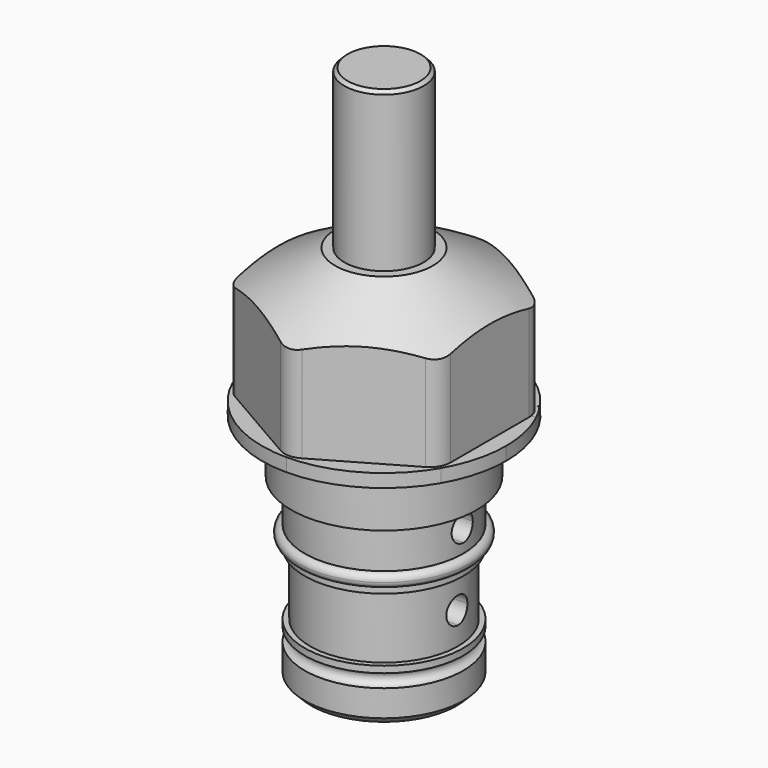
from build123d import *

# Parameters (mm, degrees)
F0_R     = 7.9375
F1_DEPTH = 35.56
F2_DEPTH = 3.175
F3_R     = 5.08
F7_SIZE  = 1.5875
F9_DEPTH = 29.3303937748
F10_W    = 9.525
F10_H    = 37.465
F10_W_2  = 3.175
F10_W_3  = 12.7
F10_H_2  = 22.606
F13_SIZE = 0.79375


with BuildPart() as f1:
    # F0 (on Top) → F1 (new body)
    with BuildSketch(Plane.XY):
        Polygon((25.4, -14.6646968374), (25.4, 14.6646968374), (0, 29.3293936748), (-25.4, 14.6646968374), (-25.4, -14.6646968374), (0, -29.3293936748), align=None)
        Circle(F0_R, mode=Mode.SUBTRACT)
        Circle(F0_R)
    extrude(amount=F1_DEPTH)

    # F0 (on Top) → F2 (join)
    with BuildSketch(Plane.XY):
        with BuildLine():
            ThreePointArc((-25.4, -14.6646968374), (-14.6646968374, -25.4), (0, -29.3293936748))
            Line((0, -29.3293936748), (-25.4, -14.6646968374))
        make_face()
        with BuildLine():
            ThreePointArc((0, -29.3293936748), (14.6646968374, -25.4), (25.4, -14.6646968374))
            Line((25.4, -14.6646968374), (0, -29.3293936748))
        make_face()
        with BuildLine():
            ThreePointArc((25.4, -14.6646968374), (28.3300188199, -7.5910056644), (29.3293936748, 0))
            ThreePointArc((29.3293936748, 0), (28.3300188199, 7.5910056644), (25.4, 14.6646968374))
            Line((25.4, 14.6646968374), (25.4, -14.6646968374))
        make_face()
        Polygon((25.4, -14.6646968374), (25.4, 14.6646968374), (0, 29.3293936748), (-25.4, 14.6646968374), (-25.4, -14.6646968374), (0, -29.3293936748), align=None)
        Circle(F0_R, mode=Mode.SUBTRACT)
        with BuildLine():
            Line((0, 29.3293936748), (25.4, 14.6646968374))
            ThreePointArc((25.4, 14.6646968374), (14.6646968374, 25.4), (0, 29.3293936748))
        make_face()
        with BuildLine():
            Line((-25.4, 14.6646968374), (0, 29.3293936748))
            ThreePointArc((0, 29.3293936748), (-14.6646968374, 25.4), (-25.4, 14.6646968374))
        make_face()
        with BuildLine():
            Line((-25.4, -14.6646968374), (-25.4, 14.6646968374))
            ThreePointArc((-25.4, 14.6646968374), (-29.3293936748, 0), (-25.4, -14.6646968374))
        make_face()
    extrude(amount=F2_DEPTH)

    # F3 (call 1 of 6: OpenCascade refuses the feature's edges together)
    f3_edges = [f1.edges().sort_by_distance(p)[0] for p in [
        (0, -29.329394, 19.3675),
    ]]
    fillet(f3_edges, radius=F3_R)

    # F3#2 (call 2 of 6)
    f3_2_edges = [f1.edges().sort_by_distance(p)[0] for p in [
        (25.4, -14.664697, 19.3675),
    ]]
    fillet(f3_2_edges, radius=F3_R)

    # F3#3 (call 3 of 6)
    f3_3_edges = [f1.edges().sort_by_distance(p)[0] for p in [
        (25.4, 14.664697, 19.3675),
    ]]
    fillet(f3_3_edges, radius=F3_R)

    # F3#4 (call 4 of 6)
    f3_4_edges = [f1.edges().sort_by_distance(p)[0] for p in [
        (0, 29.329394, 19.3675),
    ]]
    fillet(f3_4_edges, radius=F3_R)

    # F3#5 (call 5 of 6)
    f3_5_edges = [f1.edges().sort_by_distance(p)[0] for p in [
        (-25.4, 14.664697, 19.3675),
    ]]
    fillet(f3_5_edges, radius=F3_R)

    # F3#6 (call 6 of 6)
    f3_6_edges = [f1.edges().sort_by_distance(p)[0] for p in [
        (-25.4, -14.664697, 19.3675),
    ]]
    fillet(f3_6_edges, radius=F3_R)

    # F4 (on Right) → F5 (revolve, cut)
    with BuildSketch(Plane.YZ):
        Polygon((35.3962906179, 35.56), (11.7317574699, 35.56), (35.3962906179, 21.8972754168), align=None)
    revolve(axis=Axis((0, 0, 25.9955581278), (0, 0, -1)), mode=Mode.SUBTRACT)

    # F4 (on Right) → F6 (revolve)
    with BuildSketch(Plane.YZ):
        with BuildLine():
            Line((17.78, -27.686), (0, -27.686))
            Line((0, -27.686), (0, -32.131))
            ThreePointArc((0, -32.131), (2.2450640303, -33.0609359697), (3.175, -35.306))
            ThreePointArc((3.175, -35.306), (2.2450640303, -37.5510640303), (0, -38.481))
            Line((0, -38.481), (0, -42.926))
            Line((0, -42.926), (17.78, -42.926))
            Line((17.78, -42.926), (17.78, -27.686))
        make_face()
        with BuildLine():
            Line((19.05, -12.7), (0, -12.7))
            Line((0, -12.7), (0, -14.2875))
            ThreePointArc((0, -14.2875), (2.2450640303, -15.2174359697), (3.175, -17.4625))
            ThreePointArc((3.175, -17.4625), (2.2450640303, -19.7075640303), (0, -20.6375))
            Line((0, -20.6375), (0, -27.686))
            Line((0, -27.686), (17.78, -27.686))
            Line((17.78, -27.686), (19.05, -27.686))
            Line((19.05, -27.686), (19.05, -26.0985))
            ThreePointArc((19.05, -26.0985), (17.4625, -24.511), (19.05, -22.9235))
            Line((19.05, -22.9235), (19.05, -12.7))
        make_face()
        Polygon((22.225, 0), (0, 0), (0, -12.7), (19.05, -12.7), (22.225, -12.7), align=None)
        with BuildLine():
            Line((19.05, -42.926), (17.78, -42.926))
            Line((17.78, -42.926), (0, -42.926))
            Line((0, -42.926), (0, -55.626))
            Line((0, -55.626), (19.05, -55.626))
            Line((19.05, -55.626), (19.05, -47.6885))
            ThreePointArc((19.05, -47.6885), (17.4625, -46.101), (19.05, -44.5135))
            Line((19.05, -44.5135), (19.05, -42.926))
        make_face()
    revolve(axis=Axis((0, 0, 25.9955581278), (0, 0, -1)))

    # F7
    f7_edges = [f1.edges().sort_by_distance(p)[0] for p in [
        (0, -19.05, -55.626),
    ]]
    chamfer(f7_edges, length=F7_SIZE)


with BuildPart() as f8:
    # F4 (on Right) → F8 (revolve)
    with BuildSketch(Plane.YZ):
        with BuildLine():
            Line((0, -20.6375), (0, -14.2875))
            ThreePointArc((0, -14.2875), (-3.175, -17.4625), (0, -20.6375))
        make_face()
    revolve(axis=Axis((0, 0, 25.9955581278), (0, 0, -1)))


with BuildPart() as f8b:
    # F4 (on Right) → F8, piece 2 (revolve)
    with BuildSketch(Plane.YZ):
        with BuildLine():
            ThreePointArc((20.6375, -24.511), (20.1725320151, -23.3884679849), (19.05, -22.9235))
            Line((19.05, -22.9235), (19.05, -26.0985))
            ThreePointArc((19.05, -26.0985), (20.1725320151, -25.6335320151), (20.6375, -24.511))
        make_face()
        with BuildLine():
            Line((19.05, -26.0985), (19.05, -22.9235))
            ThreePointArc((19.05, -22.9235), (17.4625, -24.511), (19.05, -26.0985))
        make_face()
    revolve(axis=Axis((0, 0, 25.9955581278), (0, 0, -1)))


with BuildPart() as f9_tool:
    # F4 (on Right) → F9 (new body, through all)
    with BuildSketch(Plane.YZ):
        with BuildLine():
            Line((0, -20.6375), (0, -14.2875))
            ThreePointArc((0, -14.2875), (-3.175, -17.4625), (0, -20.6375))
        make_face()
        with BuildLine():
            ThreePointArc((3.175, -17.4625), (2.2450640303, -15.2174359697), (0, -14.2875))
            Line((0, -14.2875), (0, -20.6375))
            ThreePointArc((0, -20.6375), (2.2450640303, -19.7075640303), (3.175, -17.4625))
        make_face()
        with BuildLine():
            Line((0, -38.481), (0, -32.131))
            ThreePointArc((0, -32.131), (-3.175, -35.306), (0, -38.481))
        make_face()
        with BuildLine():
            ThreePointArc((3.175, -35.306), (2.2450640303, -33.0609359697), (0, -32.131))
            Line((0, -32.131), (0, -38.481))
            ThreePointArc((0, -38.481), (2.2450640303, -37.5510640303), (3.175, -35.306))
        make_face()
    extrude(amount=F9_DEPTH)


with BuildPart() as f1_1:
    add(f1.part)

    # F9: cut by f9_tool
    add(f9_tool.part, mode=Mode.SUBTRACT)


with BuildPart() as f8_1:
    add(f8.part)

    # F9: cut by f9_tool
    add(f9_tool.part, mode=Mode.SUBTRACT)


with BuildPart() as f11_tool:
    # F10 (on Right) → F11 (revolve)
    with BuildSketch(Plane.YZ):
        Polygon((9.525, 73.66), (0, 73.66), (0, 15.875), (9.525, 15.875), (9.525, 21.374261314), align=None)
        Polygon((9.525, 21.374261314), (9.525, 15.875), (12.7, 15.875), align=None)
        with Locations((4.7625, -2.8575)):
            Rectangle(F10_W, F10_H)
        with Locations((11.1125, -2.8575)):
            Rectangle(F10_W_2, F10_H)
        with Locations((6.35, -39.243)):
            Rectangle(F10_W_3, F10_H_2)
        Polygon((9.525, -21.59), (0, -21.59), (0, -27.94), (12.7, -27.94), (12.7, -21.59), align=None)
    revolve(axis=Axis((0, 0, 11.557), (0, 0, -1)))


with BuildPart() as f1_2:
    add(f1_1.part)

    # F11: cut by f11_tool
    add(f11_tool.part, mode=Mode.SUBTRACT)


with BuildPart() as f8_2:
    add(f8_1.part)

    # F11: cut by f11_tool
    add(f11_tool.part, mode=Mode.SUBTRACT)


with BuildPart() as f12:
    # F10 (on Right) → F12 (revolve)
    with BuildSketch(Plane.YZ):
        Polygon((9.525, 73.66), (0, 73.66), (0, 15.875), (9.525, 15.875), (9.525, 21.374261314), align=None)
        with Locations((4.7625, -2.8575)):
            Rectangle(F10_W, F10_H)
        Polygon((9.525, -21.59), (0, -21.59), (0, -27.94), (12.7, -27.94), (12.7, -21.59), align=None)
    revolve(axis=Axis((0, 0, 11.557), (0, 0, -1)))

    # F13
    f13_edges = [f12.edges().sort_by_distance(p)[0] for p in [
        (0, -9.525, 73.66),
    ]]
    chamfer(f13_edges, length=F13_SIZE)


with BuildPart() as f14_1:
    # F14: copy of F8b
    add(f8b.part)


solid = Compound([f8b.part, f1_2.part, f12.part, f14_1.part])
